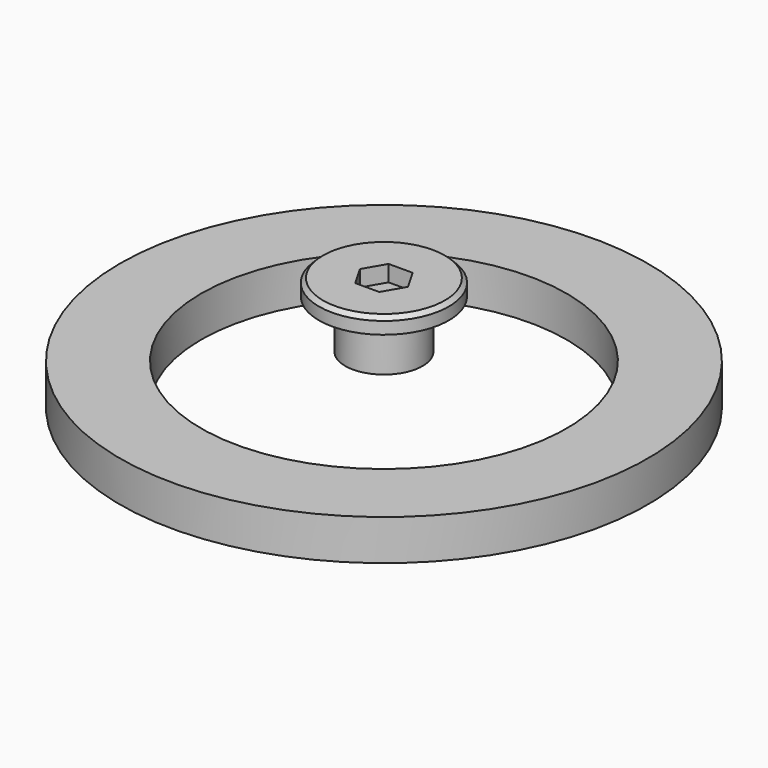
from build123d import *

# Parameters (mm, degrees)
F0_W     = 0.79375
F0_H     = 4.5
F3_DEPTH = 2
F4_SIZE  = 0.5
F0_W_2   = 7.754
F0_H_2   = 5
F0_W_3   = 2.246


# Not quite as in the source:
# - a feature of the source that left no trace in its solid (it failed there, or was rolled back) is left out


with BuildPart() as f1:
    # F0 (on Front) → F1 (revolve)
    with BuildSketch(Plane.XZ):
        Polygon((-3.96875, -3.5), (-3.96875, -8), (0, -8), (0, 0), (-8, 0), (-8, -2), (-6, -2), (-3.96875, -2), (-3.96875, -2.5), align=None)
        with Locations((-4.365625, -5.75)):
            Rectangle(F0_W, F0_H)
    revolve(axis=Axis((0, 0, -5.6257829033), (0, 0, 1)))

    # F2 (on face) → F3 (cut)
    with BuildSketch(Plane.XY):
        Polygon((1.4794600648, 2.5625), (-1.4794600648, 2.5625), (-2.9589201296, 0), (-1.4794600648, -2.5625), (1.4794600648, -2.5625), (2.9589201296, 0), align=None)
    extrude(amount=-F3_DEPTH, mode=Mode.SUBTRACT)

    # F4
    f4_edges = [f1.edges().sort_by_distance(p)[0] for p in [
        (8, 0, 0),
    ]]
    chamfer(f4_edges, length=F4_SIZE)


with BuildPart() as f6:
    # F0 (on Front) → F6 (revolve)
    with BuildSketch(Plane.XZ):
        with Locations((-26.377, -11.5)):
            Rectangle(F0_W_2, F0_H_2)
        with Locations((-31.377, -11.5)):
            Rectangle(F0_W_3, F0_H_2)
    revolve(axis=Axis((0, 0, -5.6257829033), (0, 0, 1)))


solid = Compound([f1.part, f6.part])
